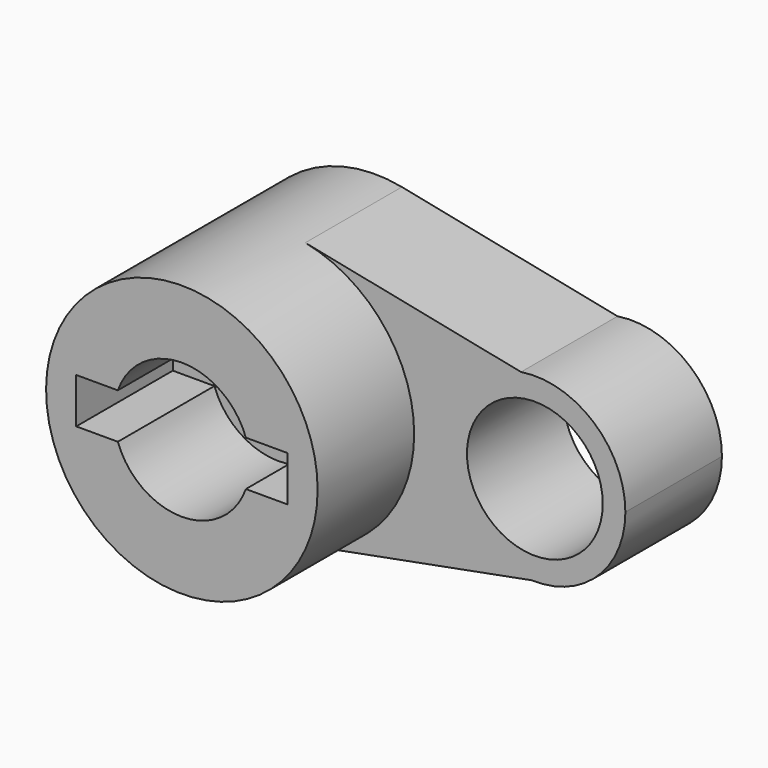
from build123d import *

# Parameters (mm, degrees)
F0_R     = 14.2875
F1_DEPTH = 25.4
F2_DEPTH = 25.4
F3_DEPTH = 50.8


with BuildPart() as f1:
    # F0 (on Front) → F1 (new body)
    with BuildSketch(Plane.XZ):
        with BuildLine():
            ThreePointArc((5.2887591577, -28.0813043068), (21.9961009946, -18.240125165), (28.575, 0))
            ThreePointArc((28.575, 0), (22.118144808, 18.0919400633), (5.6655830094, 28.0077095487))
            ThreePointArc((5.6655830094, 28.0077095487), (-28.5743551441, 0.1919716148), (5.2887591577, -28.0813043068))
        make_face()
        with BuildLine():
            ThreePointArc((-13.4703841816, 4.7625), (0, 14.2875), (13.4703841816, 4.7625))
            Line((13.4703841816, 4.7625), (22.225, 4.7625))
            Line((22.225, 4.7625), (22.225, -4.7625))
            Line((22.225, -4.7625), (13.4703841816, -4.7625))
            ThreePointArc((13.4703841816, -4.7625), (0, -14.2875), (-13.4703841816, -4.7625))
            Line((-13.4703841816, -4.7625), (-22.225, -4.7625))
            Line((-22.225, -4.7625), (-22.225, 4.7625))
            Line((-22.225, 4.7625), (-13.4703841816, 4.7625))
        make_face(mode=Mode.SUBTRACT)
        with BuildLine():
            ThreePointArc((73.025, 0), (66.3713381906, 14.464898875), (51.0582494002, 18.8253835536))
            ThreePointArc((51.0582494002, 18.8253835536), (34.9584276531, -1.1280408576), (53.304272269, -19.0381885775))
            ThreePointArc((53.304272269, -19.0381885775), (67.2061212058, -13.7054708652), (73.025, 0))
        make_face()
        with Locations((53.975, 0)):
            Circle(F0_R, mode=Mode.SUBTRACT)
        with BuildLine():
            ThreePointArc((5.6655830094, 28.0077095487), (22.118144808, 18.0919400633), (28.575, 0))
            ThreePointArc((28.575, 0), (21.9961009946, -18.240125165), (5.2887591577, -28.0813043068))
            Line((5.2887591577, -28.0813043068), (53.304272269, -19.0381885775))
            ThreePointArc((53.304272269, -19.0381885775), (34.9584276531, -1.1280408576), (51.0582494002, 18.8253835536))
            Line((51.0582494002, 18.8253835536), (5.6655830094, 28.0077095487))
        make_face()
        with BuildLine():
            ThreePointArc((-13.4703841816, -4.7625), (-14.2875, 0), (-13.4703841816, 4.7625))
            Line((-13.4703841816, 4.7625), (-22.225, 4.7625))
            Line((-22.225, 4.7625), (-22.225, -4.7625))
            Line((-22.225, -4.7625), (-13.4703841816, -4.7625))
        make_face()
    extrude(amount=F1_DEPTH)

    # F0 (on Front) → F2 (join)
    with BuildSketch(Plane.XZ):
        with BuildLine():
            ThreePointArc((5.6655830094, 28.0077095487), (22.118144808, 18.0919400633), (28.575, 0))
            ThreePointArc((28.575, 0), (21.9961009946, -18.240125165), (5.2887591577, -28.0813043068))
            Line((5.2887591577, -28.0813043068), (53.304272269, -19.0381885775))
            ThreePointArc((53.304272269, -19.0381885775), (34.9584276531, -1.1280408576), (51.0582494002, 18.8253835536))
            Line((51.0582494002, 18.8253835536), (5.6655830094, 28.0077095487))
        make_face()
        with BuildLine():
            Line((-13.4703841816, 4.7625), (13.4703841816, 4.7625))
            ThreePointArc((13.4703841816, 4.7625), (0, 14.2875), (-13.4703841816, 4.7625))
        make_face()
        with BuildLine():
            ThreePointArc((-13.4703841816, -4.7625), (0, -14.2875), (13.4703841816, -4.7625))
            Line((13.4703841816, -4.7625), (-13.4703841816, -4.7625))
        make_face()
    extrude(amount=F2_DEPTH)

    # F0 (on Front) → F3 (join)
    with BuildSketch(Plane.XZ):
        with BuildLine():
            ThreePointArc((5.2887591577, -28.0813043068), (21.9961009946, -18.240125165), (28.575, 0))
            ThreePointArc((28.575, 0), (22.118144808, 18.0919400633), (5.6655830094, 28.0077095487))
            ThreePointArc((5.6655830094, 28.0077095487), (-28.5743551441, 0.1919716148), (5.2887591577, -28.0813043068))
        make_face()
        with BuildLine():
            ThreePointArc((-13.4703841816, 4.7625), (0, 14.2875), (13.4703841816, 4.7625))
            Line((13.4703841816, 4.7625), (22.225, 4.7625))
            Line((22.225, 4.7625), (22.225, -4.7625))
            Line((22.225, -4.7625), (13.4703841816, -4.7625))
            ThreePointArc((13.4703841816, -4.7625), (0, -14.2875), (-13.4703841816, -4.7625))
            Line((-13.4703841816, -4.7625), (-22.225, -4.7625))
            Line((-22.225, -4.7625), (-22.225, 4.7625))
            Line((-22.225, 4.7625), (-13.4703841816, 4.7625))
        make_face(mode=Mode.SUBTRACT)
    extrude(amount=F3_DEPTH)


solid = f1.part
